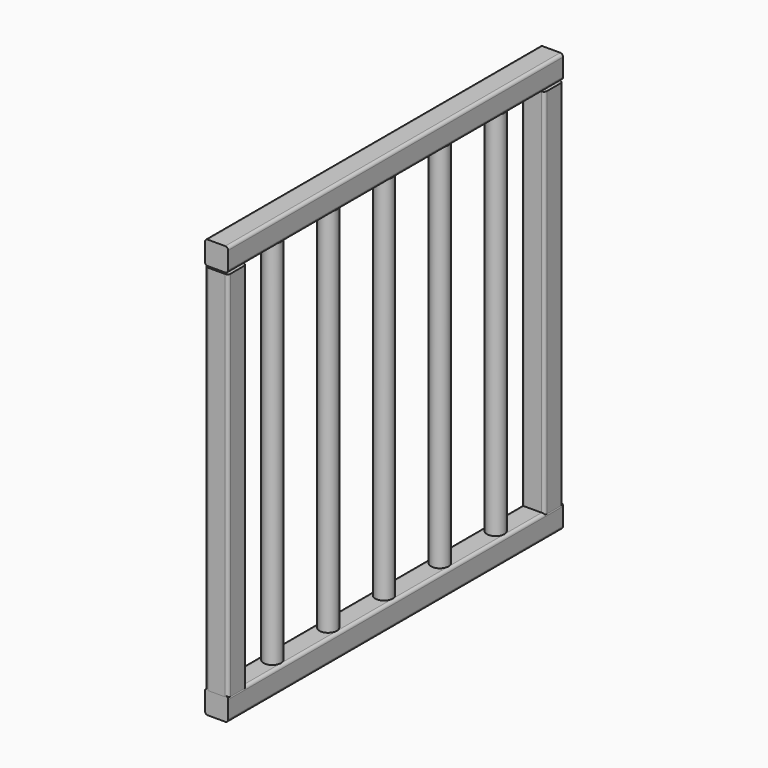
from build123d import *

# Parameters (mm, degrees)
F1_DEPTH = 914.4
F3_R     = 19.05
F4_DEPTH = 812.8


with BuildPart() as f1:
    # F0 (on Front) → F1 (new body)
    with BuildSketch(Plane.XZ):
        with BuildLine():
            Line((-19.05, 84.0507361742), (19.05, 84.0507361742))
            ThreePointArc((19.05, 84.0507361742), (23.5401280605, 85.9106081136), (25.4, 90.4007361742))
            Line((25.4, 90.4007361742), (25.4, 128.5007361742))
            ThreePointArc((25.4, 128.5007361742), (23.5401280605, 132.9908642347), (19.05, 134.8507361742))
            Line((19.05, 134.8507361742), (-19.05, 134.8507361742))
            ThreePointArc((-19.05, 134.8507361742), (-23.5401280605, 132.9908642347), (-25.4, 128.5007361742))
            Line((-25.4, 128.5007361742), (-25.4, 90.4007361742))
            ThreePointArc((-25.4, 90.4007361742), (-23.5401280605, 85.9106081136), (-19.05, 84.0507361742))
        make_face()
    extrude(amount=F1_DEPTH)


with BuildPart() as f1b:
    # F0 (on Front) → F1, piece 2 (new body)
    with BuildSketch(Plane.XZ):
        with BuildLine():
            ThreePointArc((25.4, -735.0992638258), (23.5401280605, -730.6091357653), (19.05, -728.7492638258))
            Line((19.05, -728.7492638258), (-19.05, -728.7492638258))
            ThreePointArc((-19.05, -728.7492638258), (-23.5401280605, -730.6091357653), (-25.4, -735.0992638258))
            Line((-25.4, -735.0992638258), (-25.4, -773.1992638258))
            ThreePointArc((-25.4, -773.1992638258), (-23.5401280605, -777.6893918864), (-19.05, -779.5492638258))
            Line((-19.05, -779.5492638258), (19.05, -779.5492638258))
            ThreePointArc((19.05, -779.5492638258), (23.5401280605, -777.6893918864), (25.4, -773.1992638258))
            Line((25.4, -773.1992638258), (25.4, -735.0992638258))
        make_face()
    extrude(amount=F1_DEPTH)


with BuildPart() as f4:
    # F3 (on offset) → F4 (new body)
    with BuildSketch(Plane.XY.offset(81.0033306479)):
        with Locations((0, -152.4)):
            Circle(F3_R)
    extrude(amount=-F4_DEPTH)


with BuildPart() as f4b:
    # F3 (on offset) → F4, piece 2 (new body)
    with BuildSketch(Plane.XY.offset(81.0033306479)):
        with Locations((0, -304.8)):
            Circle(F3_R)
    extrude(amount=-F4_DEPTH)


with BuildPart() as f4c:
    # F3 (on offset) → F4, piece 3 (new body)
    with BuildSketch(Plane.XY.offset(81.0033306479)):
        with Locations((0, -609.6)):
            Circle(F3_R)
    extrude(amount=-F4_DEPTH)


with BuildPart() as f4d:
    # F3 (on offset) → F4, piece 4 (new body)
    with BuildSketch(Plane.XY.offset(81.0033306479)):
        with Locations((0, -762)):
            Circle(F3_R)
    extrude(amount=-F4_DEPTH)


with BuildPart() as f4e:
    # F3 (on offset) → F4, piece 5 (new body)
    with BuildSketch(Plane.XY.offset(81.0033306479)):
        with Locations((0, -457.2)):
            Circle(F3_R)
    extrude(amount=-F4_DEPTH)


with BuildPart() as f4f:
    # F3 (on offset) → F4, piece 6 (new body)
    with BuildSketch(Plane.XY.offset(81.0033306479)):
        with BuildLine():
            ThreePointArc((25.4, -6.35), (23.5401280605, -1.8598719395), (19.05, 0))
            Line((19.05, 0), (-19.05, 0))
            ThreePointArc((-19.05, 0), (-23.5401280605, -1.8598719395), (-25.4, -6.35))
            Line((-25.4, -6.35), (-25.4, -44.45))
            ThreePointArc((-25.4, -44.45), (-23.5401280605, -48.9401280605), (-19.05, -50.8))
            Line((-19.05, -50.8), (19.05, -50.8))
            ThreePointArc((19.05, -50.8), (23.5401280605, -48.9401280605), (25.4, -44.45))
            Line((25.4, -44.45), (25.4, -6.35))
        make_face()
    extrude(amount=-F4_DEPTH)


with BuildPart() as f4g:
    # F3 (on offset) → F4, piece 7 (new body)
    with BuildSketch(Plane.XY.offset(81.0033306479)):
        with BuildLine():
            ThreePointArc((25.4, -869.95), (23.5401280605, -865.4598719395), (19.05, -863.6))
            Line((19.05, -863.6), (-19.05, -863.6))
            ThreePointArc((-19.05, -863.6), (-23.5401280605, -865.4598719395), (-25.4, -869.95))
            Line((-25.4, -869.95), (-25.4, -908.05))
            ThreePointArc((-25.4, -908.05), (-23.5401280605, -912.5401280605), (-19.05, -914.4))
            Line((-19.05, -914.4), (19.05, -914.4))
            ThreePointArc((19.05, -914.4), (23.5401280605, -912.5401280605), (25.4, -908.05))
            Line((25.4, -908.05), (25.4, -869.95))
        make_face()
    extrude(amount=-F4_DEPTH)


solid = Compound([f1.part, f1b.part, f4.part, f4b.part, f4c.part, f4d.part, f4e.part, f4f.part, f4g.part])
